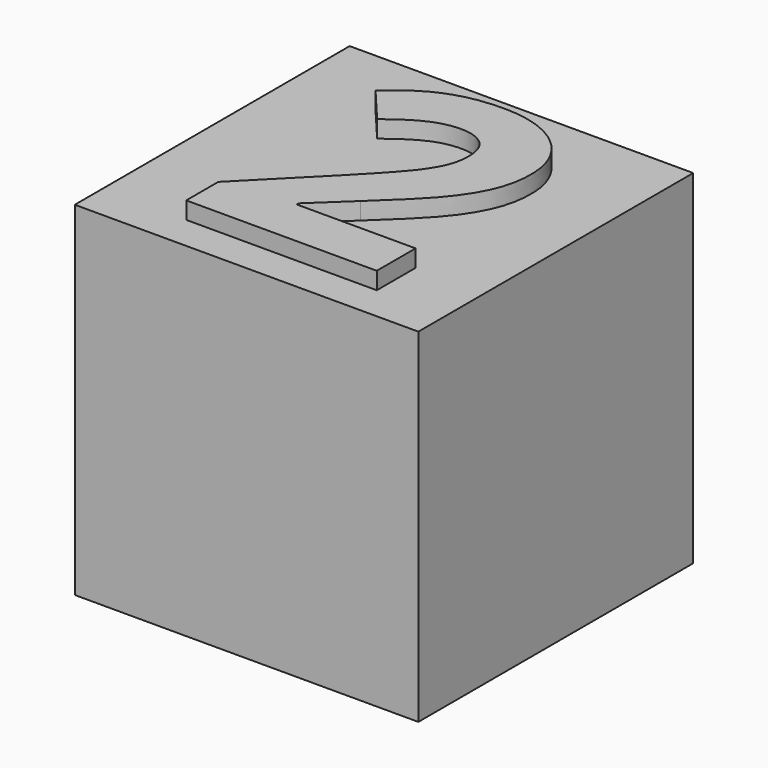
from build123d import *

# Parameters (mm, degrees)
F0_W         = 10
F0_H         = 10
F1_DEPTH     = 10
F2_TEXT_SIZE = 11.1111111111
F3_DEPTH     = 0.5


# Not quite as in the source:
# - Text() gives the source's letters only with a copy of the font that has no kerning and outlines rounded to 1/6400 em; it was checked with that copy


with BuildPart() as f1:
    # F0 (on Top) → F1 (new body)
    with BuildSketch(Plane.XY):
        with Locations((5, 5)):
            Rectangle(F0_W, F0_H)
    extrude(amount=F1_DEPTH)

    # F2 (on face) → F3 (join)
    with BuildSketch(Plane.XY.offset(10)):
        with Locations((2, 1)):
            Text('2', F2_TEXT_SIZE, font='Open Sans', font_style=FontStyle.BOLD, text_align=(TextAlign.LEFT, TextAlign.BOTTOM))
    extrude(amount=F3_DEPTH)


solid = f1.part
